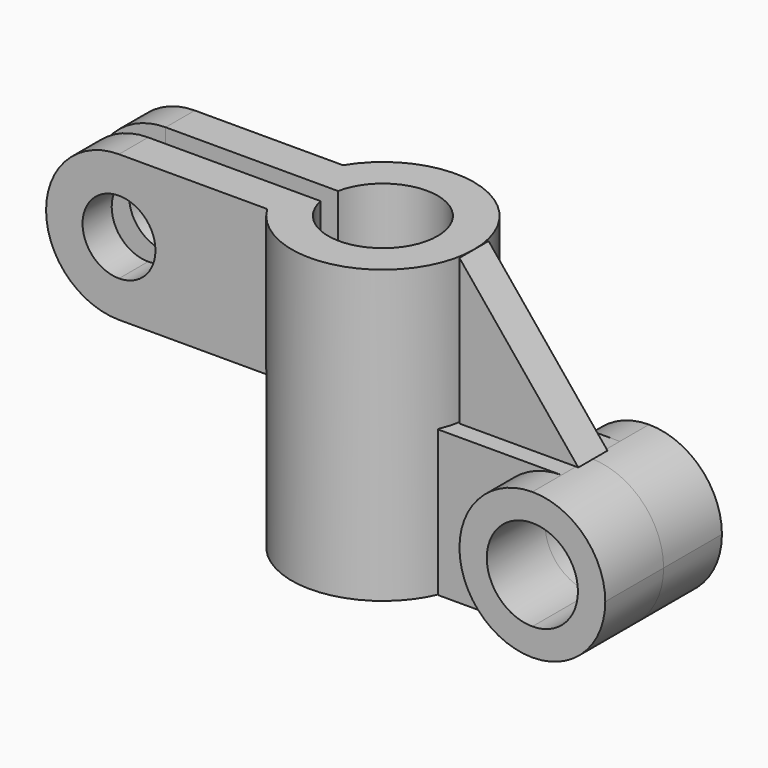
from build123d import *

# Parameters (mm, degrees)
F0_R           = 25
F0_R_2         = 15
F1_DEPTH       = 80
F3_DEPTH       = 13
F3_DEPTH_BACK  = 13
F4_DEPTH       = 4.5
F5_W           = 28.1823416352
F5_H           = 3
F6_DEPTH       = 99.3
F8_DEPTH       = 10
F8_DEPTH_BACK  = 10
F9_DEPTH       = 20
F9_DEPTH_BACK  = 20
F10_DEPTH      = 1.9
F12_DEPTH      = 5
F12_DEPTH_BACK = 5


# Not quite as in the source:
# - ends of sketch curves that miss each other by under 0.0002 mm in the source are joined


with BuildPart() as f1:
    # F0 (on Top) → F1 (new body)
    with BuildSketch(Plane.XY):
        Circle(F0_R)
        Circle(F0_R_2, mode=Mode.SUBTRACT)
    extrude(amount=F1_DEPTH)



with BuildPart() as f3:
    # F2 (on Front) → F3 (new body, two sides)
    with BuildSketch(Plane.XZ) as f3_sk:
        with BuildLine():
            Line((-62, 40), (-25, 40))
            Line((-25, 40), (-25, 80))
            Line((-25, 80), (-62, 80))
            ThreePointArc((-62, 80), (-47.8578643763, 74.1421356237), (-42, 60))
            ThreePointArc((-42, 60), (-47.8578643763, 45.8578643763), (-62, 40))
        make_face()
        with BuildLine():
            ThreePointArc((-62, 80), (-82, 60), (-62, 40))
            Line((-62, 40), (-62, 50))
            ThreePointArc((-62, 50), (-72, 60), (-62, 70))
            Line((-62, 70), (-62, 80))
        make_face()
        with BuildLine():
            Line((-62, 50), (-62, 40))
            ThreePointArc((-62, 40), (-47.8578643763, 45.8578643763), (-42, 60))
            ThreePointArc((-42, 60), (-47.8578643763, 74.1421356237), (-62, 80))
            Line((-62, 80), (-62, 70))
            ThreePointArc((-62, 70), (-54.9289321881, 67.0710678119), (-52, 60))
            ThreePointArc((-52, 60), (-54.9289321881, 52.9289321881), (-62, 50))
        make_face()
    extrude(amount=F3_DEPTH)
    extrude(f3_sk.sketch, amount=-F3_DEPTH_BACK)


with BuildPart() as f1_1:
    add(f1.part)
    # F4 (add): a face of the model
    f4_faces = [f3.part.faces().sort_by_distance(p)[0] for p in [
        (-25, 0, 60),
    ]]

    add(f3.part)  # F4 merges F3
    extrude(f4_faces, amount=F4_DEPTH)

    # F5 (on face) → F6 (cut)
    with BuildSketch(Plane.XY.offset(80)):
        Polygon((-90.1823416352, 0), (-62, 0), (-62, 2.9951323172), (-90.1823415071, 3.0011918221), align=None)
        with Locations((-76.0911708176, -1.5)):
            Rectangle(F5_W, F5_H)
        with BuildLine():
            Line((-62, 0), (-15, 0))
            ThreePointArc((-15, 0), (-14.9248115566, 1.5), (-14.7, 2.9849623113))
            Line((-14.7, 2.9849623113), (-62, 2.9951323172))
            Line((-62, 2.9951323172), (-62, 0))
        make_face()
        with BuildLine():
            ThreePointArc((-14.6969384567, -3), (-14.9240422951, -1.5076344301), (-15, 0))
            Line((-15, 0), (-62, 0))
            Line((-62, 0), (-62, -3))
            Line((-62, -3), (-14.6969384567, -3))
        make_face()
    extrude(amount=-F6_DEPTH, mode=Mode.SUBTRACT)



with BuildPart() as f8:
    # F7 (on Front) → F8 (new body, two sides)
    with BuildSketch(Plane.XZ) as f8_sk:
        with BuildLine():
            Line((57, 40), (25, 40))
            Line((25, 40), (25, 0))
            Line((25, 0), (57, 0))
            ThreePointArc((57, 0), (37, 20), (57, 40))
        make_face()
    extrude(amount=F8_DEPTH)
    extrude(f8_sk.sketch, amount=-F8_DEPTH_BACK)


with BuildPart() as f9:
    # F7 (on Front) → F9 (new body, two sides)
    with BuildSketch(Plane.XZ) as f9_sk:
        with BuildLine():
            ThreePointArc((77, 20), (71.1421356237, 34.1421356237), (57, 40))
            Line((57, 40), (57, 32.5))
            ThreePointArc((57, 32.5), (65.8388347648, 28.8388347648), (69.5, 20))
            ThreePointArc((69.5, 20), (65.8388347648, 11.1611652352), (57, 7.5))
            Line((57, 7.5), (57, 0))
            ThreePointArc((57, 0), (71.1421356237, 5.8578643763), (77, 20))
        make_face()
        with BuildLine():
            Line((57, 32.5), (57, 40))
            ThreePointArc((57, 40), (37, 20), (57, 0))
            Line((57, 0), (57, 7.5))
            ThreePointArc((57, 7.5), (44.5, 20), (57, 32.5))
        make_face()
    extrude(amount=F9_DEPTH)
    extrude(f9_sk.sketch, amount=-F9_DEPTH_BACK)


with BuildPart() as f1_2:
    add(f1_1.part)
    # F10 (add): a face of the model
    f10_faces = [f8.part.faces().sort_by_distance(p)[0] for p in [
        (25, 0, 20),
    ]]

    add(f8.part)  # F10 merges F8
    extrude(f10_faces, amount=F10_DEPTH)


with BuildPart() as f12:
    # F11 (on Front) → F12 (new body, two sides)
    with BuildSketch(Plane.XZ) as f12_sk:
        with BuildLine():
            Line((57.6036605042, 39.9908877741), (25, 80))
            Line((25, 80), (25, 40))
            Line((25, 40), (56.4075138858, 39.9912220788))
            ThreePointArc((56.4075138858, 39.9912220788), (57.0055896948, 39.9999992189), (57.6036605042, 39.9908877741))
        make_face()
    extrude(amount=F12_DEPTH)
    extrude(f12_sk.sketch, amount=-F12_DEPTH_BACK)


solid = Compound([f9.part, f1_2.part, f12.part])
